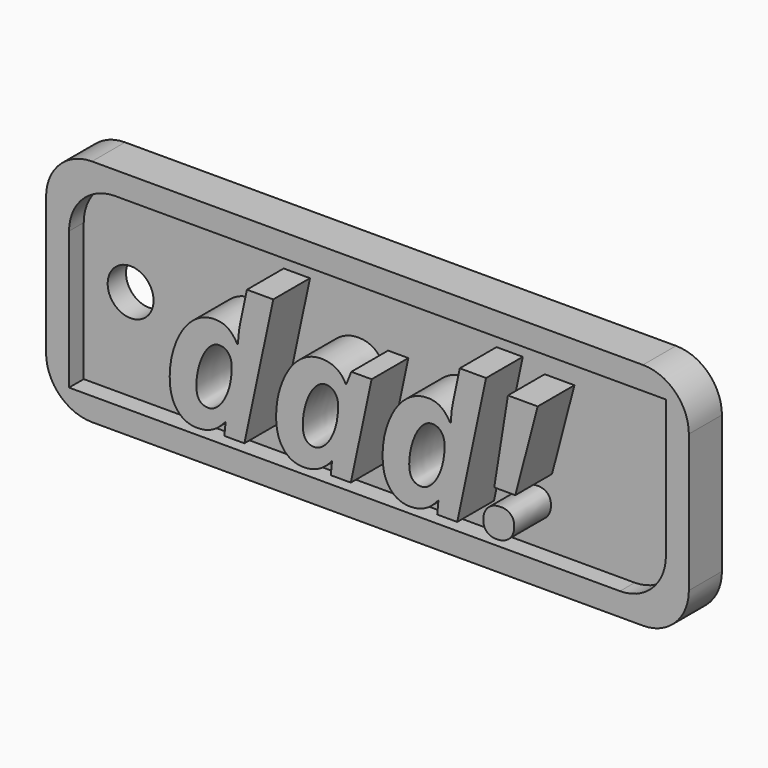
from build123d import *

# Parameters (mm, degrees)
F1_DEPTH     = 2.5
F3_DEPTH     = 2
F4_TEXT_SIZE = 19.5039352143
F5_DEPTH     = 5
F7_D         = 5


# Not quite as in the source:
# - Text() gives the source's letters only with a copy of the font that has no kerning and outlines rounded to 1/6400 em; it was checked with that copy


with BuildPart() as f1:
    # F0 (on Front) → F1 (new body)
    with BuildSketch(Plane.XZ):
        with BuildLine():
            Line((0, 20), (0, 5))
            ThreePointArc((0, 5), (1.4644660941, 1.4644660941), (5, 0))
            Line((5, 0), (65, 0))
            ThreePointArc((65, 0), (68.5355339059, 1.4644660941), (70, 5))
            Line((70, 5), (70, 20))
            ThreePointArc((70, 20), (68.5355339059, 23.5355339059), (65, 25))
            Line((65, 25), (5, 25))
            ThreePointArc((5, 25), (1.4644660941, 23.5355339059), (0, 20))
        make_face()
    extrude(amount=F1_DEPTH)

    # F2 (on face) → F3 (join)
    with BuildSketch(Plane.XZ.offset(2.5)):
        with BuildLine():
            Line((5, 0), (65, 0))
            ThreePointArc((65, 0), (68.5355339059, 1.4644660941), (70, 5))
            Line((70, 5), (70, 20))
            ThreePointArc((70, 20), (68.5355339059, 23.5355339059), (65, 25))
            Line((65, 25), (5, 25))
            ThreePointArc((5, 25), (1.4644660941, 23.5355339059), (0, 20))
            Line((0, 20), (0, 5))
            ThreePointArc((0, 5), (1.4644660941, 1.4644660941), (5, 0))
        make_face()
        with BuildLine():
            Line((67.5, 22.5), (67.5, 7.5))
            ThreePointArc((67.5, 7.5), (66.0355339059, 3.9644660941), (62.5, 2.5))
            Line((62.5, 2.5), (2.5, 2.5))
            Line((2.5, 2.5), (2.5, 17.5))
            ThreePointArc((2.5, 17.5), (3.9644660941, 21.0355339059), (7.5, 22.5))
            Line((7.5, 22.5), (67.5, 22.5))
        make_face(mode=Mode.SUBTRACT)
    extrude(amount=F3_DEPTH)

    # F4 (on face) → F5 (join)
    with BuildSketch(Plane.XZ.offset(2.5)):
        with Locations((15.006554313, 5.3693181835)):
            Text('dad!', F4_TEXT_SIZE, font='Open Sans', font_style=FontStyle.BOLDITALIC, text_align=(TextAlign.LEFT, TextAlign.BOTTOM))
    extrude(amount=F5_DEPTH)

    # F7 (through all)
    with Locations(Plane.XZ.offset(4.5)):
        with Locations((7.6057859696, 12.5)):
            Hole(F7_D / 2)


solid = f1.part
